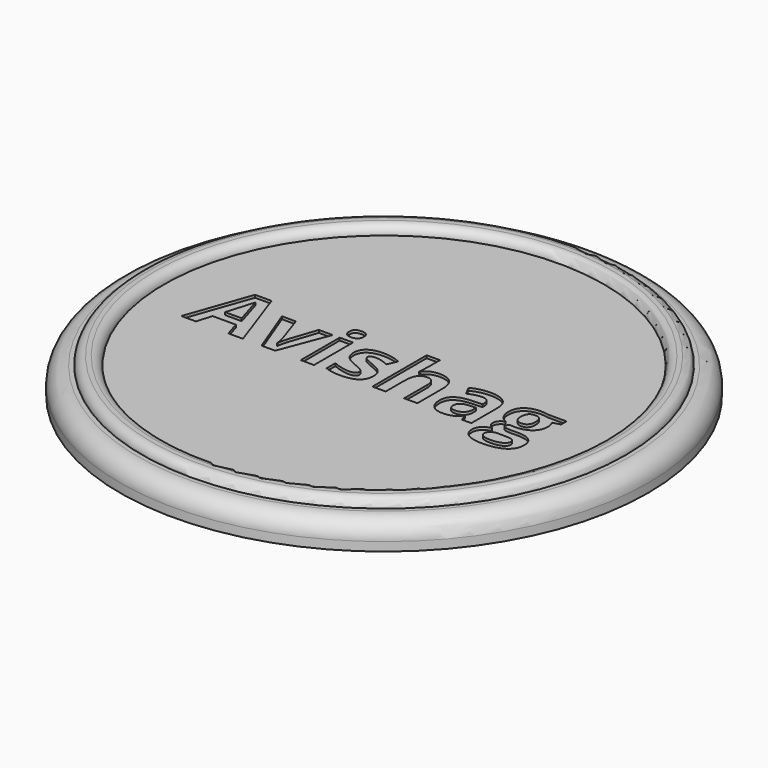
from build123d import *

# Parameters (mm, degrees)
F0_R         = 30
F0_R_2       = 27.5
F1_DEPTH     = 3
F0_R_3       = 25
F2_DEPTH     = 4
F3_R         = 2
F4_R         = 0.99999
F5_TEXT_SIZE = 10.1510765693
F6_DEPTH     = 0.3


# Not quite as in the source:
# - a fillet or chamfer is up to 0.001 mm smaller than in the source, because OpenCascade refuses the exact size
# - Text() gives the source's letters only with a copy of the font that has no kerning and outlines rounded to 1/6400 em; it was checked with that copy


with BuildPart() as f1:
    # F0 (on Top) → F1 (new body)
    with BuildSketch(Plane.XY):
        Circle(F0_R)
        Circle(F0_R_2, mode=Mode.SUBTRACT)
    extrude(amount=F1_DEPTH)



with BuildPart() as f1b:
    # F0 (on Top) → F1, piece 2 (new body)
    with BuildSketch(Plane.XY):
        Circle(F0_R_3)
    extrude(amount=F1_DEPTH)


with BuildPart() as f1_1:
    add(f1.part)

    add(f1b.part)  # F2 merges F1b
    # F0 (on Top) → F2 (join)
    with BuildSketch(Plane.XY):
        Circle(F0_R_2)
        Circle(F0_R_3, mode=Mode.SUBTRACT)
    extrude(amount=F2_DEPTH)

    # F3
    f3_edges = [f1_1.edges().sort_by_distance(p)[0] for p in [
        (-30, 0, 3),
    ]]
    fillet(f3_edges, radius=F3_R)

    # F4 (radius 1 in the source; OpenCascade refuses exactly that, so slightly less here)
    f4_edges = [f1_1.edges().sort_by_distance(p)[0] for p in [
        (-27.5, 0, 4),
        (-25, 0, 4),
    ]]
    fillet(f4_edges, radius=F4_R)

    # F5 (on face) → F6 (cut)
    with BuildSketch(Plane.XY.offset(3)):
        with Locations((-20, -3.8087751299)):
            Text('Avishag', F5_TEXT_SIZE, font='Open Sans', font_style=FontStyle.BOLD, text_align=(TextAlign.LEFT, TextAlign.BOTTOM))
    extrude(amount=-F6_DEPTH, mode=Mode.SUBTRACT)


solid = f1_1.part
